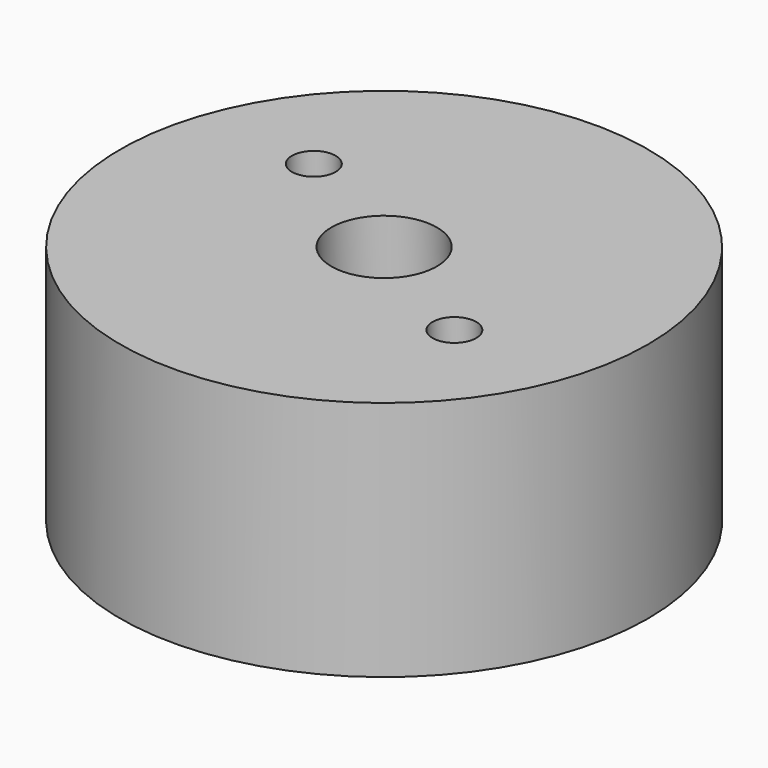
from build123d import *

# Parameters (mm, degrees)
F0_R           = 17.5
F0_R_2         = 15
F1_DEPTH       = 4
F2_DEPTH       = 12
F3_D           = 2.9
F3_CSINK_D     = 5
F3_CSINK_ANGLE = 90
F4_D           = 7


# Not quite as in the source:
# - a feature names something its author has since deleted; it is built from what else it names


with BuildPart() as f1:
    # F0 (on Top) → F1 (new body)
    with BuildSketch(Plane.XY):
        Circle(F0_R)
        Circle(F0_R_2, mode=Mode.SUBTRACT)
        Circle(F0_R_2)
    extrude(amount=F1_DEPTH)

    # F0 (on Top) → F2 (join)
    with BuildSketch(Plane.XY):
        Circle(F0_R)
        Circle(F0_R_2, mode=Mode.SUBTRACT)
    extrude(amount=-F2_DEPTH)

    # F3 (through all)
    with Locations(Plane(origin=(0, 0, 0), x_dir=(1, 0, 0), z_dir=(0, 0, -1))):
        with Locations((8.6602540378, 5), (-8.6602540378, -5)):
            CounterSinkHole(F3_D / 2, F3_CSINK_D / 2, counter_sink_angle=F3_CSINK_ANGLE)

    # F4 (through all)
    with Locations(Plane(origin=(0, 0, 0), x_dir=(1, 0, 0), z_dir=(0, 0, -1))):
        with Locations((0, 0)):
            Hole(F4_D / 2)


solid = f1.part
